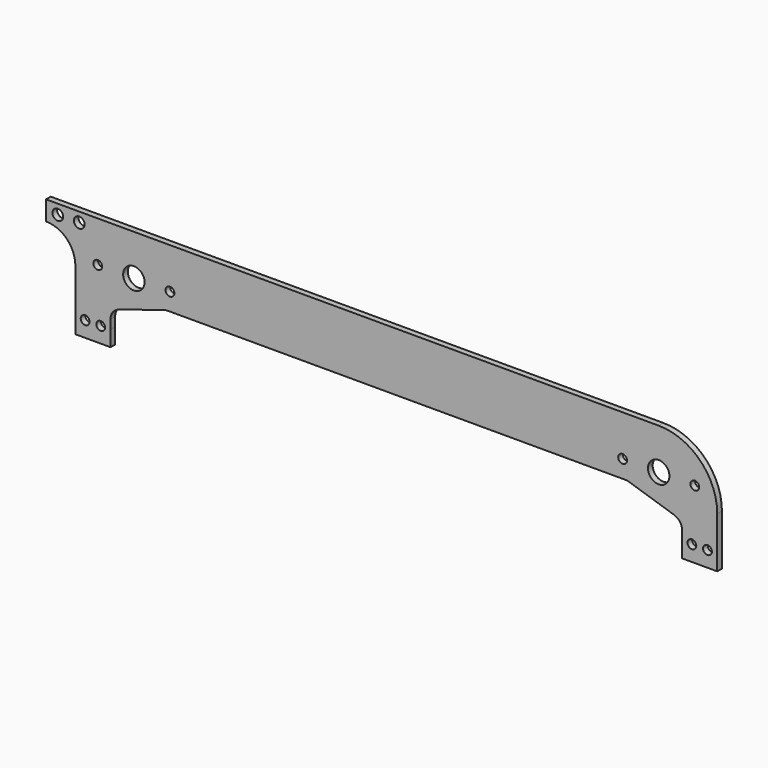
from build123d import *

# Parameters (mm, degrees)
F0_R     = 2.25
F0_R_2   = 5.5
F0_R_3   = 2.75
F1_DEPTH = 3
F2_R     = 6
F3_R     = 15


# Not quite as in the source:
# - ends of sketch curves that miss each other by under 0.0002 mm in the source are joined


with BuildPart() as f1:
    # F0 (on Front) → F1 (new body)
    with BuildSketch(Plane.XZ):
        with BuildLine():
            Line((167.4230358146, 30.0005254045), (-101.5769641849, 30.0000224371))
            ThreePointArc((-101.5769641849, 30.0000224371), (-122.790151189, 21.2131862095), (-131.576908088, -3.36535e-05))
            Line((-131.576908088, -3.36535e-05), (-131.5768594728, -26.0000336567))
            Line((-131.5768594728, -26.0000336567), (-113.5768594728, -26))
            Line((-113.5768594728, -26), (-113.5768594728, -18))
            Line((-113.5768594728, -18), (-113.57685947, -9))
            Line((-113.57685947, -9), (-113.5768594672, 0))
            Line((-113.5768594672, 0), (-85.4137075401, 0))
            Line((-85.4137075401, 0), (149.4231405226, 0))
            Line((149.4231405226, 0), (151.260137769, 0))
            Line((151.260137769, 0), (179.4231405277, -8.9999831717))
            Line((179.4231405277, -8.9999831717), (179.4231405277, -17.9999663433))
            Line((179.4231405277, -17.9999663433), (179.4231405277, -26))
            Line((179.4231405277, -26), (197.4231405276, -25.9999663433))
            Line((197.4231405276, -25.9999663433), (197.4230919114, 0.0005814952))
            ThreePointArc((197.4230919114, 0.0005814952), (188.6362556816, 21.2137685033), (167.4230358146, 30.0005254045))
        make_face()
        with Locations((-126.5768744313, -18.0000243076)):
            Circle(F0_R, mode=Mode.SUBTRACT)
        with Locations((-118.5768744313, -18.0000093491)):
            Circle(F0_R, mode=Mode.SUBTRACT)
        with Locations((184.4231255691, -17.9999663433)):
            Circle(F0_R, mode=Mode.SUBTRACT)
        with Locations((192.4231255691, -17.9999663442)):
            Circle(F0_R, mode=Mode.SUBTRACT)
        with Locations((-120.0769249193, 8.9998906191)):
            Circle(F0_R, mode=Mode.SUBTRACT)
        with Locations((-101.5769249198, 9.0000224409)):
            Circle(F0_R_2, mode=Mode.SUBTRACT)
        with Locations((-83.0769249199, 8.9999598022)):
            Circle(F0_R, mode=Mode.SUBTRACT)
        with Locations((148.9230750802, 9.0003935993)):
            Circle(F0_R, mode=Mode.SUBTRACT)
        with Locations((167.4230750797, 9.0005254008)):
            Circle(F0_R_2, mode=Mode.SUBTRACT)
        with Locations((185.9230750796, 9.0004627825)):
            Circle(F0_R, mode=Mode.SUBTRACT)
        with BuildLine():
            ThreePointArc((-131.576908088, -3.36535e-05), (-122.790151189, 21.2131862095), (-101.5769641849, 30.0000224371))
            Line((-101.5769641849, 30.0000224371), (-146.5769641849, 29.999966344))
            Line((-146.5769641849, 29.999966344), (-146.5769517198, 19.999966344))
            Line((-146.5769517198, 19.999966344), (-131.576908088, 19.999966344))
            Line((-131.576908088, 19.999966344), (-131.576908088, -3.36535e-05))
        make_face()
        with Locations((-140.5769579523, 24.999966344)):
            Circle(F0_R_3, mode=Mode.SUBTRACT)
        with Locations((-129.5769910358, 25.0335049432)):
            Circle(F0_R_3, mode=Mode.SUBTRACT)
        Polygon((-113.5768594672, 0), (-113.57685947, -9), (-85.4137075401, 0), align=None)
    extrude(amount=F1_DEPTH)

    # F2
    f2_edges = [f1.edges().sort_by_distance(p)[0] for p in [
        (-113.576859, -1.5, -9),
        (-85.413708, -1.5, 0),
        (151.260138, -1.5, 0),
        (179.423141, -1.5, -8.999983),
    ]]
    fillet(f2_edges, radius=F2_R)

    # F3
    f3_edges = [f1.edges().sort_by_distance(p)[0] for p in [
        (-131.576908, -1.5, 19.999966),
    ]]
    fillet(f3_edges, radius=F3_R)


solid = f1.part
